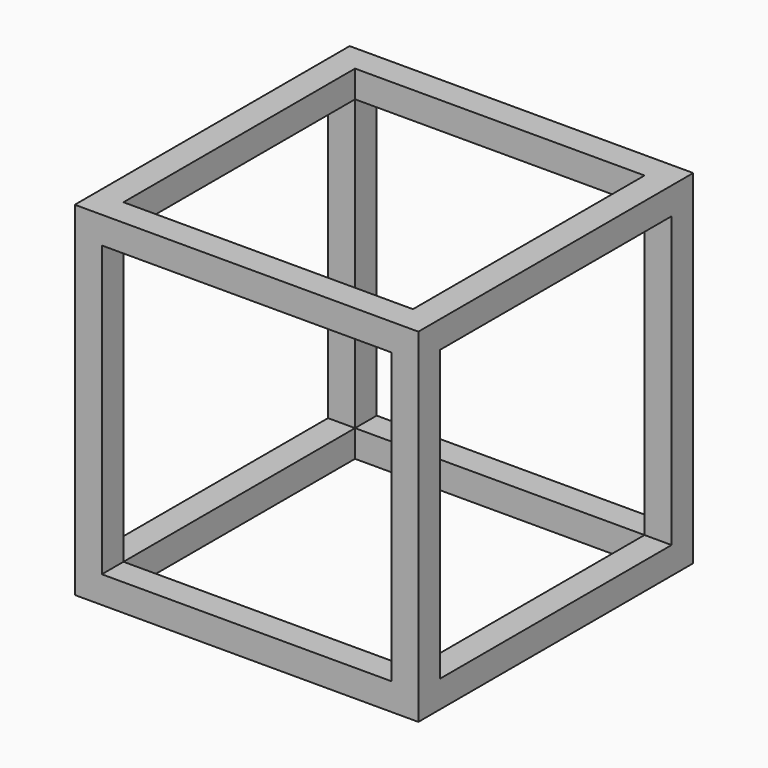
from build123d import *

# Parameters (mm, degrees)
F0_W     = 25.4
F0_H     = 25.4
F0_W_2   = 21.4
F0_H_2   = 21.4
F1_DEPTH = 25.4
F2_W     = 21.4
F2_H     = 21.4
F3_DEPTH = 25.401


# Not quite as in the source:
# - a pattern or mirror of a feature is missing from the dataset's text; its kind, count and spacing are read off the source's solid


with BuildPart() as f1:
    # F0 (on Top) → F1 (new body)
    with BuildSketch(Plane.XY):
        Rectangle(F0_W, F0_H)
        Rectangle(F0_W_2, F0_H_2, mode=Mode.SUBTRACT)
    extrude(amount=F1_DEPTH)

    # F2 (on face) → F3 (cut, through all)
    with BuildSketch(Plane.XZ.offset(12.7)):
        with Locations((0, 12.7)):
            Rectangle(F2_W, F2_H)
    f3 = extrude(amount=-F3_DEPTH, mode=Mode.SUBTRACT)

    # F3_copies: F3 across plane
    add(f3.mirror(Plane(origin=(0, 0, 0), x_dir=(-0.7071067812, 0.7071067812, 0), z_dir=(-0.7071067812, -0.7071067812, 0))), mode=Mode.SUBTRACT)


solid = f1.part
